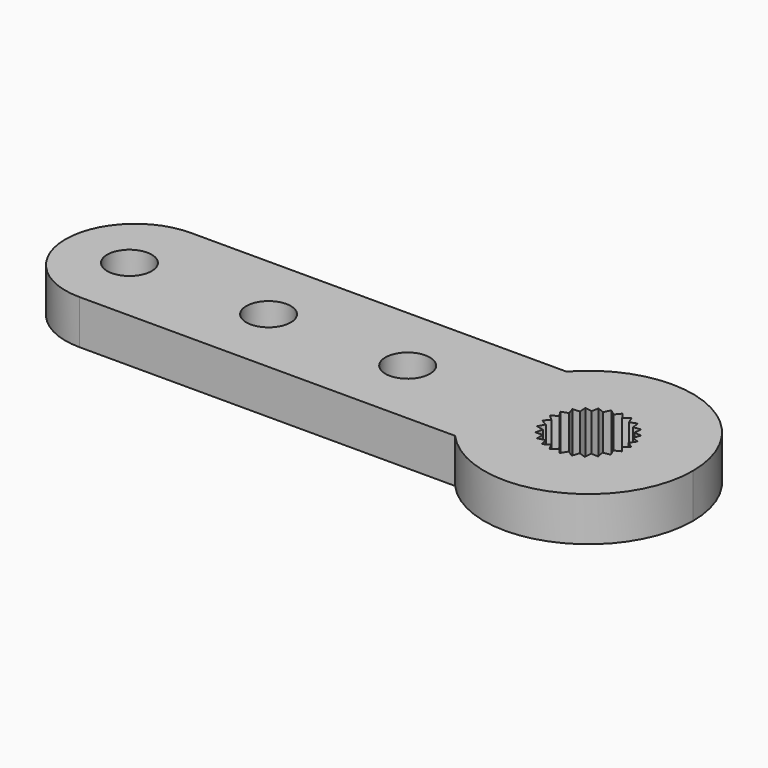
from build123d import *

# Parameters (mm, degrees)
F0_R     = 1.6
F1_DEPTH = 3.175


with BuildPart() as f1:
    # F0 (on Top) → F1 (new body)
    with BuildSketch(Plane.XY):
        with BuildLine():
            ThreePointArc((7.5, 0), (2.6761656733, 7.0062926922), (-5.5901699437, 5))
            Line((-5.5901699437, 5), (-32.6, 5))
            ThreePointArc((-32.6, 5), (-36.1355339059, 3.5355339059), (-37.6, 0))
            ThreePointArc((-37.6, 0), (-36.1355339059, -3.5355339059), (-32.6, -5))
            Line((-32.6, -5), (-5.5901699437, -5))
            ThreePointArc((-5.5901699437, -5), (2.6761656733, -7.0062926922), (7.5, 0))
        make_face()
        with Locations((-33, 0)):
            Circle(F0_R, mode=Mode.SUBTRACT)
        with Locations((-23, 0)):
            Circle(F0_R, mode=Mode.SUBTRACT)
        with Locations((-13, 0)):
            Circle(F0_R, mode=Mode.SUBTRACT)
        Polygon((-2.3131272616, 1.150841372), (-2.4811892868, 1.651717782), (-1.9542535042, 1.6899369317), (-1.992472654, 2.2168727143), (-1.4725868119, 2.1228475389), (-1.3785616365, 2.6427333809), (-0.8983920744, 2.4223718279), (-0.6780305213, 2.90254139), (-0.2677480588, 2.5696895861), (0.0651037451, 2.9799720486), (0.379719552, 2.555544297), (0.8041473037, 2.8701601039), (1.0033279869, 2.380824761), (1.4926633298, 2.5800054442), (1.5638936344, 2.0565092492), (2.0873898293, 2.1277395538), (2.0261940932, 1.6029756981), (2.5509579489, 1.5417799619), (2.3611813253, 1.0487212884), (2.8542399989, 0.8589446648), (2.547806851, 0.4285718633), (2.9781796525, 0.1221387154), (2.574344302, -0.2185063082), (2.9149893256, -0.6223416587), (2.4391262327, -0.8518549247), (2.6686394987, -1.3277180175), (2.1506488918, -1.4316783634), (2.2546092377, -1.9496689703), (1.7270383715, -1.9215441851), (1.6989135863, -2.4491150513), (1.1949116786, -2.2906723188), (1.0364689461, -2.7946742265), (0.5877042905, -2.5158690862), (0.3088991502, -2.9646337418), (-0.0564307197, -2.5829845462), (-0.4380799154, -2.9483144161), (-0.6970199802, -2.4878015876), (-1.1575328087, -2.7467416524), (-1.2938129119, -2.2363009057), (-1.8042536586, -2.3725810089), (-1.80931082, -1.8442852134), (-2.3376066155, -1.8493423749), (-2.2111230752, -1.3363862984), (-2.7240791517, -1.209902758), (-2.4740023355, -0.7445173173), (-2.9393877762, -0.4944405012), (-2.5814309304, -0.105867575), (-2.9700038565, 0.2520892708), (-2.5266587261, 0.5394342163), (-2.8140036716, 0.9827793468), align=None, mode=Mode.SUBTRACT)
    extrude(amount=F1_DEPTH)


solid = f1.part
